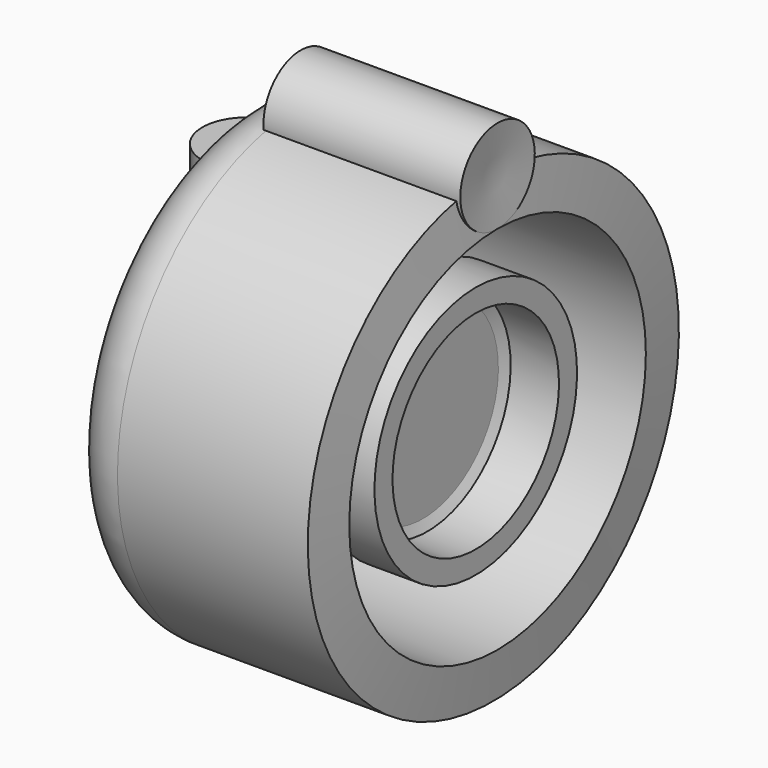
from build123d import *


# Not quite as in the source:
# - the program builds the solid bodies; features that only make, move or delete a surface that nothing else refers to are left out


with BuildPart() as f1:
    # F0 (on Front) → F1 (revolve)
    with BuildSketch(Plane.XZ):
        Polygon((0, 30.0858486444), (0, 0), (7.5085829012, 0), (7.5085829012, 30.0714652985), align=None)
    revolve(axis=Axis((0, 0, 15.0429243222), (0, 0, 1)))


with BuildPart() as f2:
    # F0 (on Front) → F2 (revolve)
    with BuildSketch(Plane.XZ):
        Polygon((41.4511226118, 39.0248671174), (9.4205942005, 39.0248671174), (9.0265786275, 31.1927329749), (42.1604327857, 31.1927329749), align=None)
    revolve(axis=Axis((25.4358584061, 0, 39.0248671174), (1, 0, 0)))


with BuildPart() as f4:
    # F0 (on Front) → F4 (revolve)
    with BuildSketch(Plane.XZ):
        Polygon((25.6762634963, 15.8565379679), (25.6762634963, 0), (29.6170078218, 0), (29.6170078218, 15.8565379679), (30.3619299084, 17.5078306347), (38.4891740978, 17.5078306347), (38.4891740978, 21.3095918298), (29.6170078218, 21.3095918298), align=None)
    revolve(axis=Axis((27.646635659, 0, 0), (-1, 0, 0)))


with BuildPart() as f4b:
    # F0 (on Front) → F4, piece 2 (revolve)
    with BuildSketch(Plane.XZ):
        Polygon((0, 30.0858486444), (0, 0), (7.5085829012, 0), (7.5085829012, 30.0714652985), align=None)
        Polygon((41.4511226118, 39.0248671174), (9.4205942005, 39.0248671174), (9.0265786275, 31.1927329749), (42.1604327857, 31.1927329749), align=None)
        with BuildLine():
            ThreePointArc((9.4205942005, 39.0248671174), (2.7899273364, 36.5791845812), (0, 30.0858486444))
            Line((0, 30.0858486444), (7.5085829012, 30.0714652985))
            ThreePointArc((7.5085829012, 30.0714652985), (7.9846999977, 31.015069059), (9.0265786275, 31.1927329749))
            Line((9.0265786275, 31.1927329749), (9.4205942005, 39.0248671174))
        make_face()
    revolve(axis=Axis((27.646635659, 0, 0), (-1, 0, 0)))


solid = Compound([f1.part, f2.part, f4.part, f4b.part])
